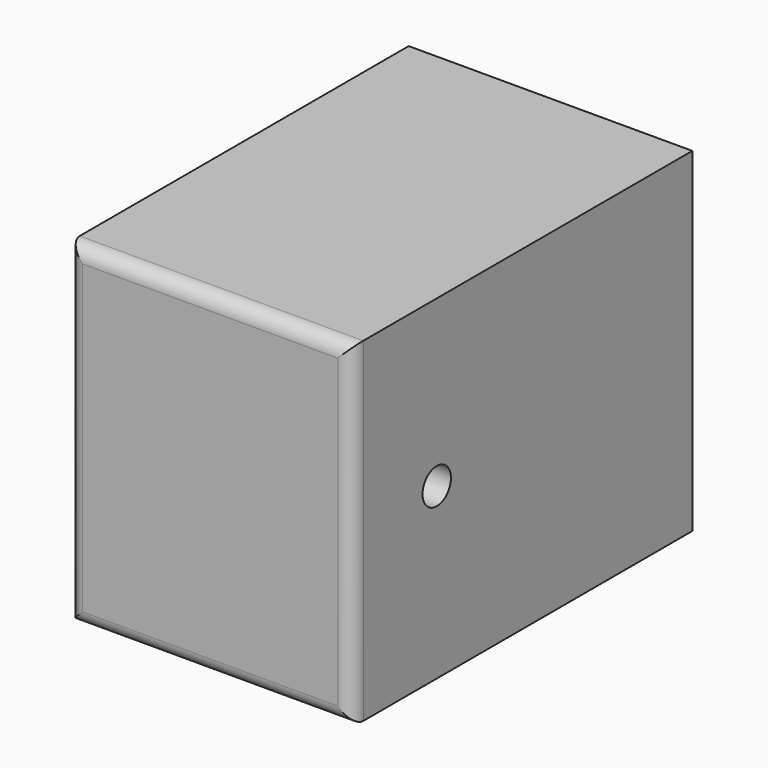
from build123d import *

# Parameters (mm, degrees)
F0_W         = 50.8
F0_H         = 59.944
F1_DEPTH     = 76.2
F2_R         = 2.54
F4_D         = 6.35
F5_TEXT_SIZE = 21.8600818092
F6_DEPTH     = 25.4


# Not quite as in the source:
# - Text() gives the source's letters only with a copy of the font that has no kerning and outlines rounded to 1/6400 em; it was checked with that copy


with BuildPart() as f1:
    # F0 (on Front) → F1 (new body)
    with BuildSketch(Plane.XZ):
        with Locations((-0.824008137, 9.0656069367)):
            Rectangle(F0_W, F0_H)
    extrude(amount=F1_DEPTH)

    # F2
    f2_edges = [f1.edges().sort_by_distance(p)[0] for p in [
        (-0.824008, -76.2, 39.037607),
        (-26.224008, -76.2, 9.065607),
        (-0.824008, -76.2, -20.906393),
        (24.575992, -76.2, 9.065607),
    ]]
    fillet(f2_edges, radius=F2_R)

    # F4 (through all)
    with Locations(Plane.YZ.offset(24.575991863)):
        with Locations((-57.220466435, 9.4398017973)):
            Hole(F4_D / 2)

    # F5 (on face) → F6 (cut)
    with BuildSketch(Plane(origin=(0, 0, 0), x_dir=(-1, 0, 0), z_dir=(0, 1, 0))):
        with Locations((-17.2282439198, 1.644937729)):
            Text('Rat', F5_TEXT_SIZE, font='Open Sans', text_align=(TextAlign.LEFT, TextAlign.BOTTOM))
    extrude(amount=-F6_DEPTH, mode=Mode.SUBTRACT)


solid = f1.part
